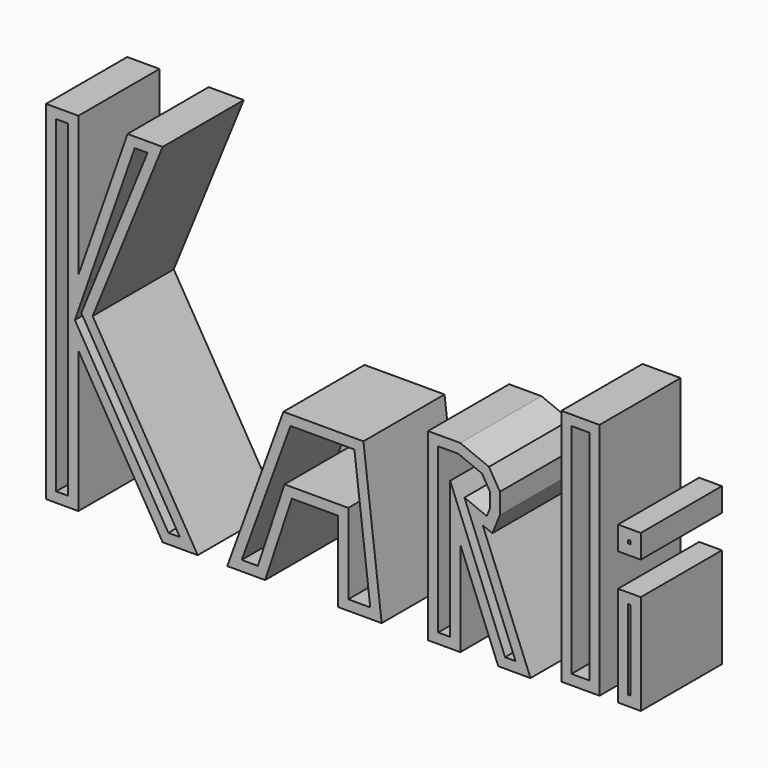
from build123d import *

# Parameters (mm, degrees)
F1_DEPTH    = 25.4
F0_W        = 9.557787329
F0_H        = 59.7195103765
F0_W_2      = 5.7009607553
F0_H_2      = 25.0989235938
F0_H_3      = 5.8975424618
F2_T        = -2.54
F3_T        = -2.54
F4_T        = -2.54
F5_T        = 2.54
F5_T3_DEPTH = 30.48
F6_T        = -2.54
F6_2_T      = -2.54


# Not quite as in the source:
# - a shell that OpenCascade refuses in one call is made with other operations: the cavity is built on its own and cut out


with BuildPart() as f1:
    # F0 (on Front) → F1 (new body)
    with BuildSketch(Plane.XZ):
        Polygon((-69.7978138924, 67.0073106885), (-69.7978138924, -20.1488938183), (-61.7104172707, -20.1488938183), (-61.7104172707, 15.2386100963), (-61.7104172707, 31.8665504456), (-61.7104172707, 67.0073106885), align=None)
        Polygon((-61.7104172707, 31.8665504456), (-61.7104172707, 15.2386100963), (-58.1411987634, 23.9966676942), (-40.6128391623, 67.0073106885), (-49.4034960866, 67.0073106885), align=None)
        Polygon((-58.1411987634, 23.9966676942), (-61.7104172707, 15.2386100963), (-40.6128391623, -20.1488938183), (-31.8221785128, -20.1488938183), align=None)
    extrude(amount=F1_DEPTH)

    # F5: shell of thickness 2.54, made by hand


with BuildPart() as f1b:
    # F0 (on Front) → F1, piece 2 (new body)
    with BuildSketch(Plane.XZ):
        Polygon((9.6697267145, 18.4547863901), (-10.3729721159, 18.4547863901), (-24.4380254298, -20.1488938183), (-14.944116585, -20.1488938183), (-8.2632154226, 0), (3.3404529095, 0), (3.3404529095, -20.1488938183), (14.2408590764, -20.1488938183), align=None)
    extrude(amount=F1_DEPTH)

    # F2
    f2_openings = [f1b.faces().sort_by_distance(p)[0] for p in [
        (-0.351623, -25.4, 17.908316),
    ]]
    offset(amount=F2_T, openings=f2_openings, kind=Kind.INTERSECTION)


with BuildPart() as f1c:
    # F0 (on Front) → F1, piece 3 (new body)
    with BuildSketch(Plane.XZ):
        Polygon((25.8445329964, 25.9793000181), (25.8445329964, 18.4547863901), (25.8445329964, 6.7574218847), (25.8445329964, -20.1488938183), (33.931940794, -20.1488938183), (33.931940794, 3.6146529019), (43.4258431196, -20.1488938183), (51.5132546425, -20.1488938183), (39.5579561591, 9.6612665802), (41.9525803864, 8.6853724377), (43.8503899663, 13.3421693182), (43.8503899663, 18.4547863901), (41.1078936159, 23.0548452138), (33.931940794, 25.9793000181), align=None)
    extrude(amount=F1_DEPTH)

    # F4
    f4_openings = [f1c.faces().sort_by_distance(p)[0] for p in [
        (35.185702, -25.4, 2.749804),
    ]]
    offset(amount=F4_T, openings=f4_openings, kind=Kind.INTERSECTION)


with BuildPart() as f1d:
    # F0 (on Front) → F1, piece 4 (new body)
    with BuildSketch(Plane.XZ):
        with Locations((64.0123244375, 11.4447139204)):
            Rectangle(F0_W, F0_H)
    extrude(amount=F1_DEPTH)

    # F3
    f3_openings = [f1d.faces().sort_by_distance(p)[0] for p in [
        (64.012324, -25.4, 11.444714),
    ]]
    offset(amount=F3_T, openings=f3_openings)


with BuildPart() as f1e:
    # F0 (on Front) → F1, piece 5 (new body)
    with BuildSketch(Plane.XZ):
        with Locations((76.2748867273, -5.865579471)):
            Rectangle(F0_W_2, F0_H_2)
    extrude(amount=F1_DEPTH)

    # F6
    f6_openings = [f1e.faces().sort_by_distance(p)[0] for p in [
        (76.274887, -25.4, -5.865579),
    ]]
    offset(amount=F6_T, openings=f6_openings)


with BuildPart() as f1f:
    # F0 (on Front) → F1, piece 6 (new body)
    with BuildSketch(Plane.XZ):
        with Locations((76.2748867273, 17.8892137483)):
            Rectangle(F0_W_2, F0_H_3)
    extrude(amount=F1_DEPTH)

    # F6#2
    f6_2_openings = [f1f.faces().sort_by_distance(p)[0] for p in [
        (76.274887, -25.4, 17.889214),
    ]]
    offset(amount=F6_2_T, openings=f6_2_openings)


with BuildPart() as f5_core1:
    # F5_t2: copy of F1
    add(f1.part)

    # the walls: a layer under each face that stays
    f5_faces = [f5_core1.faces().sort_by_distance(p)[0] for p in [
        (-69.7978138924, -12.7, 23.4292084351),
        (-65.7541155815, -12.7, -20.1488938183),
        (-61.7104172707, -12.7, -2.455141861),
        (-51.1616282165, -12.7, -2.455141861),
        (-36.2175088376, -12.7, -20.1488938183),
        (-44.9816886381, -12.7, 1.923886938),
        (-49.3770189629, -12.7, 45.5019891914),
        (-45.0081676245, -12.7, 67.0073106885),
        (-55.5569566786, -12.7, 49.436930567),
        (-61.7104172707, -12.7, 49.436930567),
        (-65.7541155815, -12.7, 67.0073106885),
        (-63.4685413291, 0, -5.6228597338),
    ]]
    thicken(f5_faces, amount=-F5_T, mode=Mode.SUBTRACT)

    # F5_s4 → F5_t3 (cut)
    with BuildSketch(Plane.XZ.offset(-2.54)):
        Polygon((-61.7068342034, 15.2256031195), (-64.2504172707, 15.2386100963), (-64.2504172707, 24.4591238986), (-59.5287239963, 16.5393077769), align=None)
        Polygon((-58.0958601368, 24.0000887481), (-60.3228920378, 22.6959700136), (-60.9710486864, 23.7831396319), (-60.493368149, 24.9552599859), align=None)
        Polygon((-61.7089896442, 31.8749459985), (-59.3131799199, 31.0269951562), (-64.2504172707, 16.9293771238), (-64.2504172707, 31.8665504456), align=None)
    extrude(amount=F5_T3_DEPTH, mode=Mode.SUBTRACT)


with BuildPart() as f1_1:
    add(f1.part)

    # what is left inside the walls is the cavity
    f5_cavity = [f5_core1.part.solids().sort_by_distance(p)[0] for p in [
        (-67.232414, -17.78, 23.429208),
        (-48.330086, -17.78, 2.530531),
    ]]
    add(f5_cavity, mode=Mode.SUBTRACT)


solid = Compound([f1b.part, f1c.part, f1d.part, f1e.part, f1f.part, f1_1.part])
